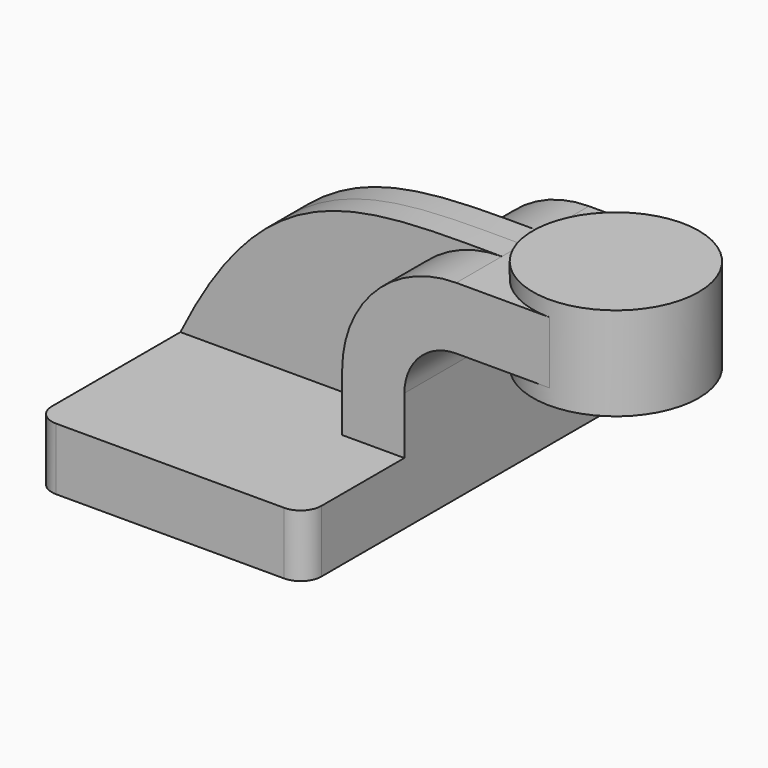
from build123d import *

# Parameters (mm, degrees)
F1_DEPTH = 63.5
F2_DEPTH = 25.4
F3_DEPTH = 7.9375
F5_R     = 6.35


with BuildPart() as f1:
    # F0 (on Front) → F1 (new body, symmetric)
    with BuildSketch(Plane.XZ):
        Polygon((-41.275, 9.525), (-41.275, -9.525), (41.275, -9.525), (41.275, 9.525), (22.225, 9.525), align=None)
    extrude(amount=F1_DEPTH, both=True)

    # F0 (on Front) → F2 (join, symmetric)
    with BuildSketch(Plane.XZ):
        with BuildLine():
            Line((22.225, 9.525), (41.275, 9.525))
            Line((41.275, 9.525), (41.275, 27.0002))
            ThreePointArc((41.275, 27.0002), (45.9246798487, 38.2255201513), (57.15, 42.8752))
            Line((57.15, 42.8752), (60.325, 42.8752))
            Line((60.325, 42.8752), (60.325, 61.9118876984))
            add(Edge.make_bspline(
                [(57.15, 61.9252), (58.2024017722, 61.9212196773), (59.2640962396, 61.9177081997), (60.325, 61.9118876984)],
                knots=[0.7123833019, 0.7123833019, 0.7123833019, 0.7123833019, 0.7293225906, 0.7293225906, 0.7293225906, 0.7293225906], degree=3))
            ThreePointArc((57.15, 61.9252), (32.4542956671, 51.6959043329), (22.225, 27.0002))
            Line((22.225, 27.0002), (22.225, 9.525))
        make_face()
        with BuildLine():
            Line((60.325, 61.9252), (57.15, 61.9252))
            add(Edge.make_bspline(
                [(57.15, 61.9252), (58.2024017722, 61.9212196773), (59.2640962396, 61.9177081997), (60.325, 61.9118876984)],
                knots=[0.7123833019, 0.7123833019, 0.7123833019, 0.7123833019, 0.7293225906, 0.7293225906, 0.7293225906, 0.7293225906], degree=3))
            Line((60.325, 61.9118876984), (60.325, 61.9252))
        make_face()
        Polygon((85.725, 61.9252), (60.325, 61.9252), (60.325, 61.9118876984), (60.325, 42.8752), (85.725, 42.8752), align=None)
    extrude(amount=F2_DEPTH, both=True)

    # F0 (on Front) → F3 (join, symmetric)
    with BuildSketch(Plane.XZ):
        with BuildLine():
            add(Edge.make_bspline(
                [(-41.275, 9.525), (-14.9323567748, 63.0891993642), (12.8911493683, 62.0925928269), (57.15, 61.9252)],
                knots=[0, 0, 0, 0, 0.7123833019, 0.7123833019, 0.7123833019, 0.7123833019], degree=3))
            Line((-41.275, 9.525), (22.225, 9.525))
            Line((22.225, 9.525), (22.225, 27.0002))
            ThreePointArc((22.225, 27.0002), (32.4542956671, 51.6959043329), (57.15, 61.9252))
        make_face()
    extrude(amount=F3_DEPTH, both=True)

    # F0 (on Front) → F4 (revolve)
    with BuildSketch(Plane.XZ):
        Polygon((85.725, 66.675), (85.725, 61.9252), (85.725, 42.8752), (85.725, 38.1), (111.125, 38.1), (111.125, 66.675), align=None)
    revolve(axis=Axis((85.725, 0, 52.3875), (0, 0, 1)))

    # F5
    f5_edges = [f1.edges().sort_by_distance(p)[0] for p in [
        (-41.275, -63.5, 0),
        (41.275, -63.5, 0),
        (41.275, 63.5, 0),
        (-41.275, 63.5, 0),
    ]]
    fillet(f5_edges, radius=F5_R)


solid = f1.part
